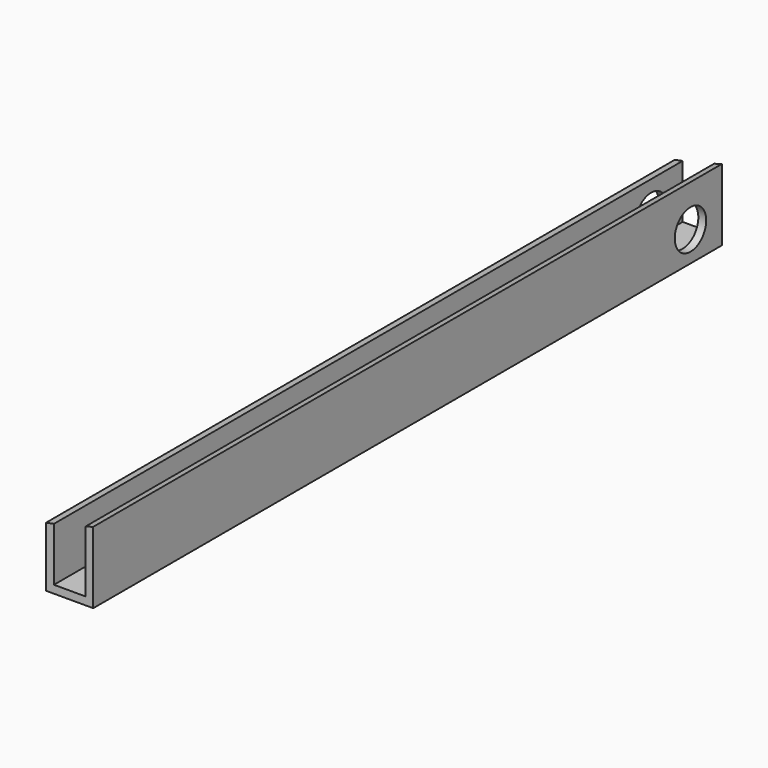
from build123d import *

# Parameters (mm, degrees)
F1_DEPTH = 500
F2_R     = 12.5
F3_DEPTH = 800


with BuildPart() as f1:
    # F0 (on Front) → F1 (new body)
    with BuildSketch(Plane.XZ):
        with BuildLine():
            Line((-14.9053066795, 14.2646563623), (-14.9053066795, -23.9014003186))
            Line((-14.9053066795, -23.9014003186), (-9.9053066795, -23.9014003186))
            Line((-9.9053066795, -23.9014003186), (-9.9053066795, -18.9014003186))
            Line((-9.9053066795, -18.9014003186), (-9.9053066795, 15.2477810018))
            ThreePointArc((-9.9053066795, 15.2477810018), (-12.4029455615, 14.7442104491), (-14.9053066795, 14.2646563623))
        make_face()
        Polygon((-9.9053066795, -18.9014003186), (-9.9053066795, -23.9014003186), (10.0946933205, -23.9014003186), (10.0946933205, -18.9014003186), (9.9053066795, -18.9014003186), align=None)
        with BuildLine():
            Line((10.0946933205, -18.9014003186), (10.0946933205, -23.9014003186))
            Line((10.0946933205, -23.9014003186), (14.9053066795, -23.9014003186))
            Line((14.9053066795, -23.9014003186), (15.0946933205, -23.9014003186))
            Line((15.0946933205, -23.9014003186), (15.0946933205, 21.6965085553))
            ThreePointArc((15.0946933205, 21.6965085553), (12.5983814298, 20.9346436244), (10.0946933205, 20.1973803878))
            Line((10.0946933205, 20.1973803878), (10.0946933205, -18.9014003186))
        make_face()
    extrude(amount=F1_DEPTH)

    # F2 (on face) → F3 (cut)
    with BuildSketch(Plane(origin=(-14.9053066795, 0, 0), x_dir=(0, -1, 0), z_dir=(-1, 0, 0))):
        with Locations((25, -4.8183719781)):
            Circle(F2_R)
    extrude(amount=-F3_DEPTH, mode=Mode.SUBTRACT)


solid = f1.part
